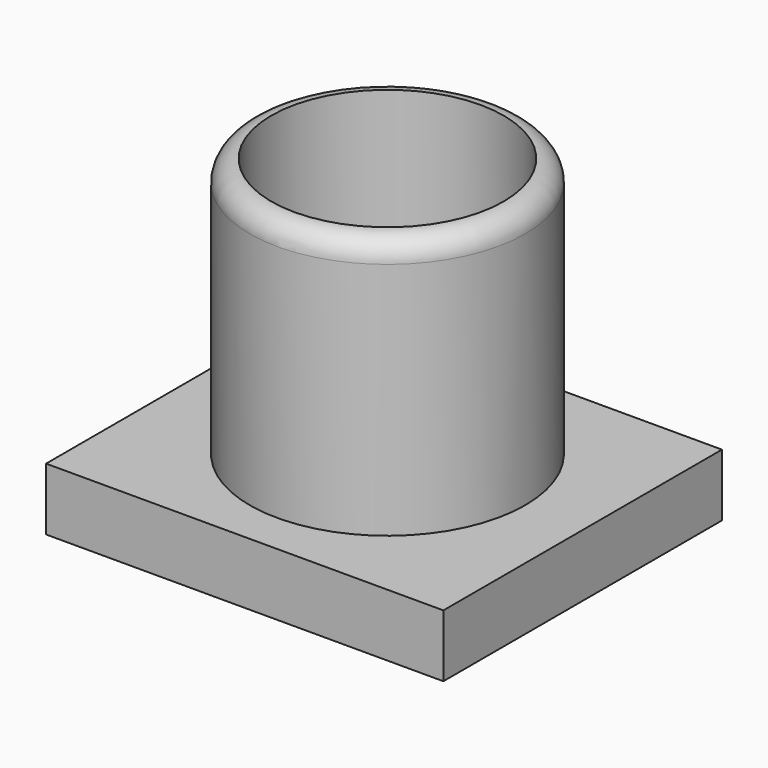
from build123d import *

# Parameters (mm, degrees)
F0_R     = 32.5185756137
F1_DEPTH = 76.2
F2_R     = 5.08
F3_DEPTH = 124.714
F4_R     = 5.07999
F5_W     = 93.7804728746
F5_H     = 82.1867324412
F6_DEPTH = 14.732
F7_DEPTH = 36.83
F8_R     = 3.4460553294
F9_DEPTH = 19.558


# Not quite as in the source:
# - a fillet or chamfer is up to 0.001 mm smaller than in the source, because OpenCascade refuses the exact size


with BuildPart() as f1:
    # F0 (on Top) → F1 (new body)
    with BuildSketch(Plane.XY):
        Circle(F0_R)
    extrude(amount=F1_DEPTH)

    # F2
    f2_edges = [f1.edges().sort_by_distance(p)[0] for p in [
        (-32.518576, 0, 76.2),
    ]]
    fillet(f2_edges, radius=F2_R)

    # F3 (cut): a face of the model
    f3_faces = [f1.faces().sort_by_distance(p)[0] for p in [
        (0, 0, 76.2),
    ]]
    extrude(f3_faces, amount=-F3_DEPTH, mode=Mode.SUBTRACT)

    # F4 (radius 5.08 in the source; OpenCascade refuses exactly that, so slightly less here)
    f4_edges = [f1.edges().sort_by_distance(p)[0] for p in [
        (-32.518576, 0, 0),
    ]]
    fillet(f4_edges, radius=F4_R)

    # F5 (on Top) → F6 (join)
    with BuildSketch(Plane.XY):
        with Locations((0.0669173896, -1.1091846973)):
            Rectangle(F5_W, F5_H)
    extrude(amount=F6_DEPTH)

    # F7 (cut): a face of the model
    f7_faces = [f1.faces().sort_by_distance(p)[0] for p in [
        (0, 0, 14.732),
    ]]
    extrude(f7_faces, amount=-F7_DEPTH, mode=Mode.SUBTRACT)

    # F8 (on Top) → F9 (cut)
    with BuildSketch(Plane.XY):
        with Locations((-42.8946092725, 35.8311235905)):
            Circle(F8_R)
    extrude(amount=F9_DEPTH, mode=Mode.SUBTRACT)


solid = f1.part
